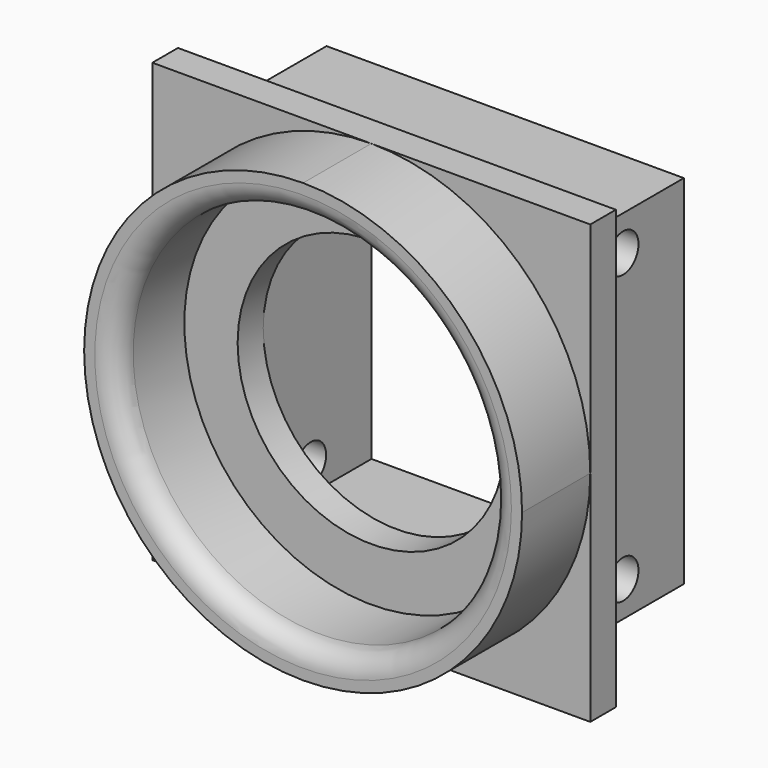
from build123d import *

# Parameters (mm, degrees)
F0_R     = 17.54425
F1_DEPTH = 3
F0_R_2   = 12.54425
F2_DEPTH = 3
F3_DEPTH = 11
F4_R     = 2
F5_W     = 33.528
F5_H     = 33.528
F5_W_2   = 3.41975
F5_H_2   = 31.928
F6_DEPTH = 12.7
F7_R     = 1.8
F8_DEPTH = 37.30925


with BuildPart() as f1:
    # F0 (on Front) → F1 (new body)
    with BuildSketch(Plane.XZ):
        with BuildLine():
            ThreePointArc((20.54425, 0), (14.5269784894, 14.5269784894), (0, 20.54425))
            ThreePointArc((0, 20.54425), (-14.5269785029, 14.5269784759), (-20.54425, -3.82e-08))
            ThreePointArc((-20.54425, -3.82e-08), (-14.5269784759, -14.5269785029), (0, -20.54425))
            ThreePointArc((0, -20.54425), (14.5269784894, -14.5269784894), (20.54425, 0))
        make_face()
        Circle(F0_R, mode=Mode.SUBTRACT)
        with BuildLine():
            Line((20.54425, 20.54425), (0, 20.54425))
            ThreePointArc((0, 20.54425), (14.5269784894, 14.5269784894), (20.54425, 0))
            Line((20.54425, 0), (20.54425, 20.54425))
        make_face()
        with BuildLine():
            Line((20.54425, -20.54425), (20.54425, 0))
            ThreePointArc((20.54425, 0), (14.5269784894, -14.5269784894), (0, -20.54425))
            Line((0, -20.54425), (20.54425, -20.54425))
        make_face()
        with BuildLine():
            Line((0, 20.54425), (-20.54425, 20.54425))
            Line((-20.54425, 20.54425), (-20.54425, -3.82e-08))
            ThreePointArc((-20.54425, -3.82e-08), (-14.5269785029, 14.5269784759), (0, 20.54425))
        make_face()
        with BuildLine():
            ThreePointArc((0, -20.54425), (-14.5269784759, -14.5269785029), (-20.54425, -3.82e-08))
            Line((-20.54425, -3.82e-08), (-20.54425, -20.54425))
            Line((-20.54425, -20.54425), (0, -20.54425))
        make_face()
    extrude(amount=F1_DEPTH)

    # F0 (on Front) → F2 (join)
    with BuildSketch(Plane.XZ):
        Circle(F0_R)
        Circle(F0_R_2, mode=Mode.SUBTRACT)
    extrude(amount=F2_DEPTH)

    # F0 (on Front) → F3 (join)
    with BuildSketch(Plane.XZ):
        with BuildLine():
            ThreePointArc((20.54425, 0), (14.5269784894, 14.5269784894), (0, 20.54425))
            ThreePointArc((0, 20.54425), (-14.5269785029, 14.5269784759), (-20.54425, -3.82e-08))
            ThreePointArc((-20.54425, -3.82e-08), (-14.5269784759, -14.5269785029), (0, -20.54425))
            ThreePointArc((0, -20.54425), (14.5269784894, -14.5269784894), (20.54425, 0))
        make_face()
        Circle(F0_R, mode=Mode.SUBTRACT)
    extrude(amount=F3_DEPTH)

    # F4
    f4_edges = [f1.edges().sort_by_distance(p)[0] for p in [
        (-17.54425, -11, 0),
    ]]
    fillet(f4_edges, radius=F4_R)

    # F5 (on Front) → F6 (join)
    with BuildSketch(Plane.XZ):
        Rectangle(F5_W, F5_H)
        Polygon((12.54425, 15.964), (15.964, 15.964), (15.964, -15.964), (12.54425, -15.964), (-12.54425, -15.964), (-15.964, -15.964), (-15.964, 15.964), (-12.54425, 15.964), align=None, mode=Mode.SUBTRACT)
        with Locations((14.254125, 0)):
            Rectangle(F5_W_2, F5_H_2)
        with Locations((-14.254125, 0)):
            Rectangle(F5_W_2, F5_H_2)
    extrude(amount=-F6_DEPTH)

    # F7 (on face) → F8 (cut, through all)
    with BuildSketch(Plane.YZ.offset(16.764)):
        with Locations((5.5796158184, 13.4703841816)):
            Circle(F7_R)
        with Locations((5.5796158184, -13.4703841816)):
            Circle(F7_R)
    extrude(amount=-F8_DEPTH, mode=Mode.SUBTRACT)


solid = f1.part
